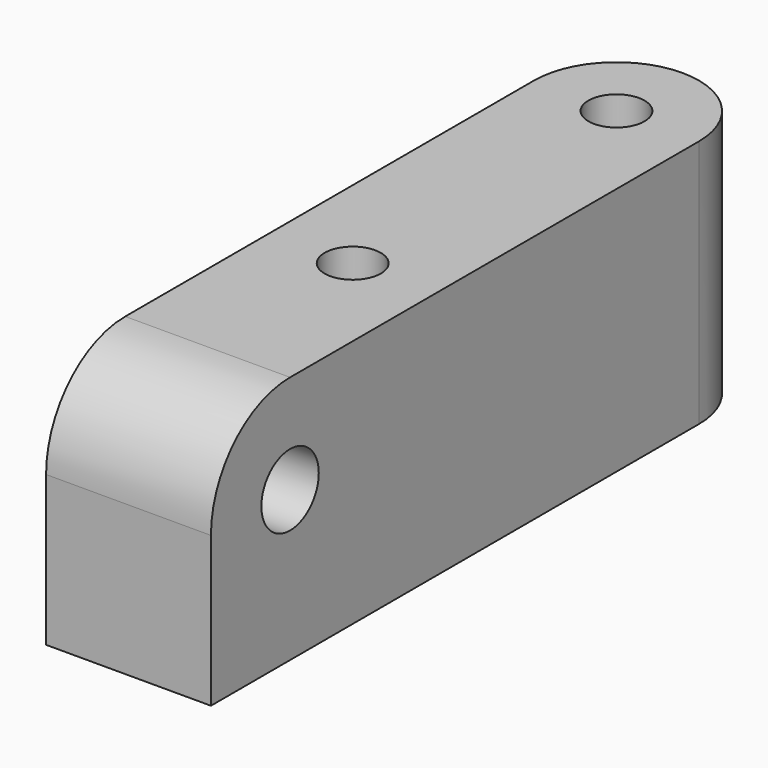
from build123d import *

# Parameters (mm, degrees)
F0_W     = 7.9375
F0_H     = 33.3375
F0_R     = 1.35255
F1_DEPTH = 11.9827929
F2_R     = 3.96874
F3_R     = 4.7625
F4_R     = 1.7272
F5_DEPTH = 7.9375
F6_R     = 3.175
F6_R_2   = 1.7272
F8_DEPTH = 4.7625


# Not quite as in the source:
# - a fillet or chamfer is up to 0.001 mm smaller than in the source, because OpenCascade refuses the exact size


with BuildPart() as f1:
    # F0 (on Top) → F1 (new body)
    with BuildSketch(Plane.XY):
        with Locations((3.96875, 16.66875)):
            Rectangle(F0_W, F0_H)
        with Locations((3.96875, 13.49375)):
            Circle(F0_R, mode=Mode.SUBTRACT)
        with Locations((3.96875, 29.36875)):
            Circle(F0_R, mode=Mode.SUBTRACT)
    extrude(amount=F1_DEPTH)

    # F2 (radius 3.96875 in the source; OpenCascade refuses exactly that, so slightly less here)
    f2_edges = [f1.edges().sort_by_distance(p)[0] for p in [
        (7.9375, 33.3375, 5.991396),
        (0, 33.3375, 5.991396),
    ]]
    fillet(f2_edges, radius=F2_R)

    # F3
    f3_edges = [f1.edges().sort_by_distance(p)[0] for p in [
        (3.96875, 0, 11.982793),
    ]]
    fillet(f3_edges, radius=F3_R)

    # F4 (on face) → F5 (cut, through all)
    with BuildSketch(Plane.YZ.offset(7.9375)):
        with Locations((4.7625, 7.2202929)):
            Circle(F4_R)
    extrude(amount=-F5_DEPTH, mode=Mode.SUBTRACT)

    # F6 (on face) → F8 (cut, through all)
    with BuildSketch(Plane(origin=(0, 0, 0), x_dir=(0, -1, 0), z_dir=(-1, 0, 0))):
        with Locations((-4.7625, 7.2202929)):
            Circle(F6_R)
        with Locations((-4.7625, 7.2202929)):
            Circle(F6_R_2, mode=Mode.SUBTRACT)
    extrude(amount=-F8_DEPTH, mode=Mode.SUBTRACT)


solid = f1.part
